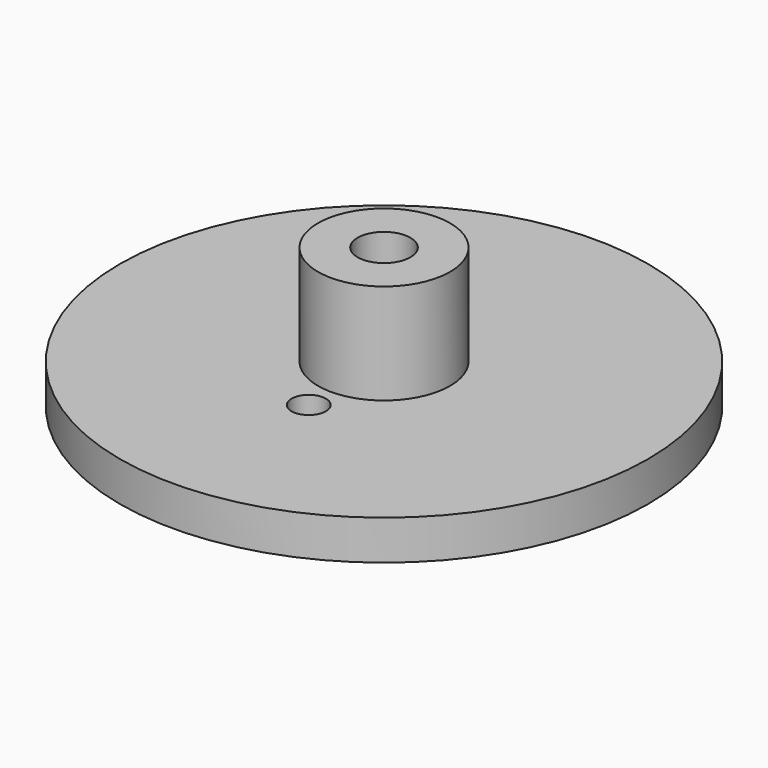
from build123d import *

# Parameters (mm, degrees)
F0_R     = 10
F0_R_2   = 1
F1_DEPTH = 1.5
F2_R     = 2.5
F2_R_2   = 1
F3_DEPTH = 3.8
F4_R     = 0.6498381819
F5_DEPTH = 1.5


# Not quite as in the source:
# - a feature names something its author has since deleted; it is built from what else it names


with BuildPart() as f1:
    # F0 (on Top) → F1 (new body)
    with BuildSketch(Plane.XY):
        Circle(F0_R)
        Circle(F0_R_2, mode=Mode.SUBTRACT)
    extrude(amount=F1_DEPTH)

    # F2 (on face) → F3 (join)
    with BuildSketch(Plane.XY.offset(1.5)):
        Circle(F2_R)
        Circle(F2_R_2, mode=Mode.SUBTRACT)
    extrude(amount=F3_DEPTH)

    # F4 (on Top) → F5 (cut, through all)
    with BuildSketch(Plane.XY):
        with Locations((0, -3.5616646055)):
            Circle(F4_R)
    extrude(amount=F5_DEPTH, mode=Mode.SUBTRACT)


solid = f1.part
